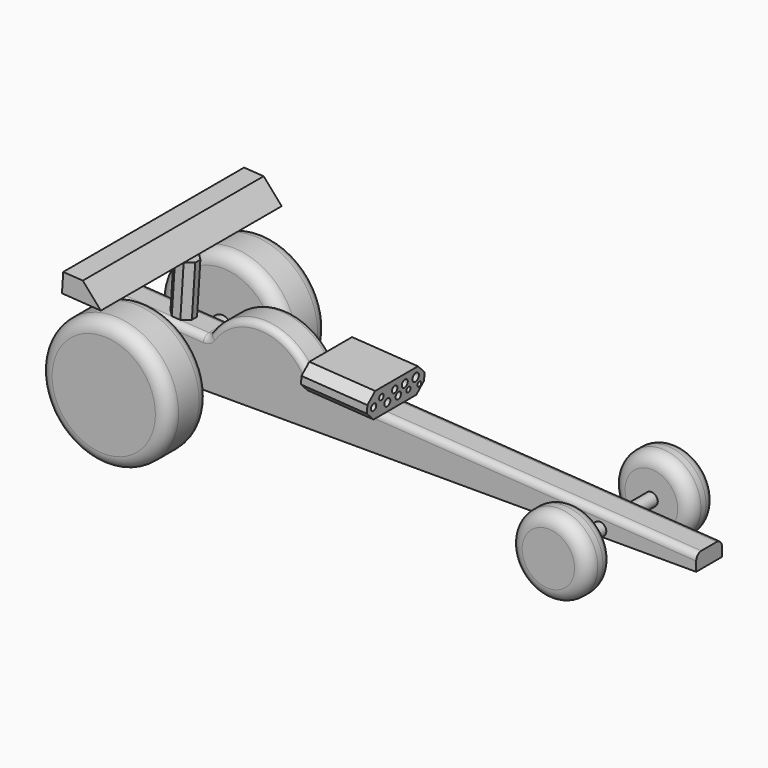
from build123d import *

# Parameters (mm, degrees)
F1_DEPTH  = 25
F2_R      = 5
F3_W      = 51.2955540023
F3_H      = 20.3379537165
F4_DEPTH  = 20
F5_SIZE   = 7
F6_R      = 2.6177928451
F6_R_2    = 2.224559375
F6_R_3    = 2.9142650528
F6_R_4    = 2.6477797202
F6_R_5    = 2.6621803072
F6_R_6    = 2.8962018761
F6_R_7    = 2.0272267168
F6_R_8    = 3.1578374874
F6_R_9    = 1.8431345388
F7_DEPTH  = 55
F8_R      = 8.0630442653
F8_R_2    = 4.9640165804
F9_DEPTH  = 25
F10_DEPTH = 50
F11_R     = 30.4357287845
F12_DEPTH = 25
F13_R     = 30.3480649607
F14_DEPTH = 25
F15_R     = 50.1181633855
F16_DEPTH = 40
F17_R     = 50.1439992572
F18_DEPTH = 40
F19_R     = 10
F20_W     = 15
F20_H     = 31.953419765
F21_DEPTH = 25
F22_W     = 16.6535501336
F22_H     = 15
F23_DEPTH = 40
F24_SIZE  = 5
F26_DEPTH = 15
F27_SIZE  = 14.99999


# Not quite as in the source:
# - a fillet or chamfer is up to 0.001 mm smaller than in the source, because OpenCascade refuses the exact size


with BuildPart() as f1:
    # F0 (on Front) → F1 (new body)
    with BuildSketch(Plane.XZ):
        Polygon((0, 41.5879301727), (0, 0), (450.1805007458, 0), (450.1805007458, 12.3640811071), (152.0178636457, 31.719561607), (70.666636126, 37.0005455465), align=None)
        with BuildLine():
            ThreePointArc((152.0178636457, 31.719561607), (112.9874016283, 59.702890297), (70.666636126, 37.0005455465))
            Line((70.666636126, 37.0005455465), (152.0178636457, 31.719561607))
        make_face()
    extrude(amount=F1_DEPTH)

    # F2
    f2_edges = [f1.edges().sort_by_distance(p)[0] for p in [
        (112.987402, -25, 59.70289),
        (112.987402, 0, 59.70289),
        (152.017864, -12.5, 31.719562),
        (301.099182, 0, 22.041821),
        (301.099182, -25, 22.041821),
        (70.666636, -12.5, 37.000546),
        (35.333318, 0, 39.294238),
        (35.333318, -25, 39.294238),
    ]]
    fillet(f2_edges, radius=F2_R)

    # F3 (on face) → F4 (join)
    with BuildSketch(Plane(origin=(2.6883867209, 0, 41.4134112683), x_dir=(0.9978996024, 0, -0.0647794991), z_dir=(0.0647794991, 0, 0.9978996024))):
        Polygon((152.6482946076, 15.1970647275), (152.6482946076, -20), (203.9438486099, -20), (203.9438486099, -5), (203.9438486099, 15.1970647275), align=None)
        with Locations((178.2960716088, -30.1689768583)):
            Rectangle(F3_W, F3_H)
    extrude(amount=F4_DEPTH)

    # F5
    f5_edges = [f1.edges().sort_by_distance(p)[0] for p in [
        (181.905556, -40.337954, 49.821473),
        (180.609966, -40.337954, 29.863481),
        (181.905556, 15.197065, 49.821473),
        (180.609966, 15.197065, 29.863481),
    ]]
    chamfer(f5_edges, length=F5_SIZE)

    # F6 (on face) → F7 (cut)
    with BuildSketch(Plane(origin=(203.5154854418, 0, -13.2113803668), x_dir=(0, 1, 0), z_dir=(0.9978996024, 0, -0.0647794991))):
        with Locations((-34.0123698115, 50.4040382802)):
            Circle(F6_R)
        with Locations((-26.718499139, 54.5005789844)):
            Circle(F6_R_2)
        with Locations((-20.4353481531, 48.1231324375)):
            Circle(F6_R_3)
        with Locations((-13.8251967728, 54.5005789844)):
            Circle(F6_R_4)
        with Locations((-9.7883678973, 48.4310872853)):
            Circle(F6_R_5)
        with Locations((-4.0084165521, 54.5005789844)):
            Circle(F6_R_6)
        with Locations((0, 48.6739836633)):
            Circle(F6_R_7)
        with Locations((6.5571470186, 54.5005789844)):
            Circle(F6_R_8)
        with Locations((10.6426598504, 48.0703115463)):
            Circle(F6_R_9)
    extrude(amount=-F7_DEPTH, mode=Mode.SUBTRACT)

    # F8 (on face) → F9 (join)
    with BuildSketch(Plane(origin=(0, 0, 0), x_dir=(-1, 0, 0), z_dir=(0, 1, 0))):
        with Locations((-42.0035384595, 14.5227285102)):
            Circle(F8_R)
        with Locations((-375.3835856915, 5.0112064928)):
            Circle(F8_R_2)
    extrude(amount=F9_DEPTH)

    # F8 (on face) → F10 (join)
    with BuildSketch(Plane(origin=(0, 0, 0), x_dir=(-1, 0, 0), z_dir=(0, 1, 0))):
        with Locations((-42.0035384595, 14.5227285102)):
            Circle(F8_R)
        with Locations((-375.3835856915, 5.0112064928)):
            Circle(F8_R_2)
    extrude(amount=-F10_DEPTH)

    # F11 (on face) → F12 (join)
    with BuildSketch(Plane(origin=(0, 25, 0), x_dir=(-1, 0, 0), z_dir=(0, 1, 0))):
        with Locations((-375.3835856915, 5.0112064928)):
            Circle(F11_R)
    extrude(amount=F12_DEPTH)

    # F13 (on face) → F14 (join)
    with BuildSketch(Plane.XZ.offset(50)):
        with Locations((375.3835856915, 5.0112064928)):
            Circle(F13_R)
    extrude(amount=F14_DEPTH)

    # F15 (on face) → F16 (join)
    with BuildSketch(Plane.XZ.offset(50)):
        with Locations((42.0035384595, 14.5227285102)):
            Circle(F15_R)
    extrude(amount=F16_DEPTH)

    # F17 (on face) → F18 (join)
    with BuildSketch(Plane(origin=(0, 25, 0), x_dir=(-1, 0, 0), z_dir=(0, 1, 0))):
        with Locations((-42.0035384595, 14.5227285102)):
            Circle(F17_R)
    extrude(amount=F18_DEPTH)

    # F19
    f19_edges = [f1.edges().sort_by_distance(p)[0] for p in [
        (92.147538, 65, 14.522729),
        (92.147538, 25, 14.522729),
        (-8.114625, -50, 14.522729),
        (-8.114625, -90, 14.522729),
        (345.035521, -75, 5.011206),
        (345.035521, -50, 5.011206),
        (405.819314, 25, 5.011206),
        (405.819314, 50, 5.011206),
    ]]
    fillet(f19_edges, radius=F19_R)

    # F20 (on face) → F21 (cut)
    with BuildSketch(Plane(origin=(0, 0, 0), x_dir=(0, -1, 0), z_dir=(-1, 0, 0))):
        with Locations((12.5, 20.6006961975)):
            Rectangle(F20_W, F20_H)
    extrude(amount=-F21_DEPTH, mode=Mode.SUBTRACT)

    # F22 (on face) → F23 (join)
    with BuildSketch(Plane(origin=(2.6883867209, 0, 41.4134112683), x_dir=(0.9978996024, 0, -0.0647794991), z_dir=(0.0647794991, 0, 0.9978996024))):
        with Locations((39.5381649507, -12.5)):
            Rectangle(F22_W, F22_H)
    extrude(amount=F23_DEPTH)

    # F24
    f24_edges = [f1.edges().sort_by_distance(p)[0] for p in [
        (35.12981, -5, 59.349545),
        (51.748381, -5, 58.270736),
        (51.748381, -20, 58.270736),
        (35.12981, -20, 59.349545),
    ]]
    chamfer(f24_edges, length=F24_SIZE)

    # F25 (on face) → F26 (join)
    with BuildSketch(Plane(origin=(5.2795666867, 0, 81.3293953647), x_dir=(0.9978996024, 0, -0.0647794991), z_dir=(0.0647794991, 0, 0.9978996024))):
        Polygon((42.8649400175, -100.4156246781), (42.8649400175, -20), (42.8649400175, -5), (42.8649400175, 75.1928910613), (12.6054044813, 75.1928910613), (12.6054044813, -100.4156246781), align=None)
    extrude(amount=F26_DEPTH)

    # F27 (size 15 in the source; OpenCascade refuses exactly that, so slightly less here)
    f27_edges = [f1.edges().sort_by_distance(p)[0] for p in [
        (49.026166, -12.611367, 93.52112),
    ]]
    chamfer(f27_edges, length=F27_SIZE)


solid = f1.part
